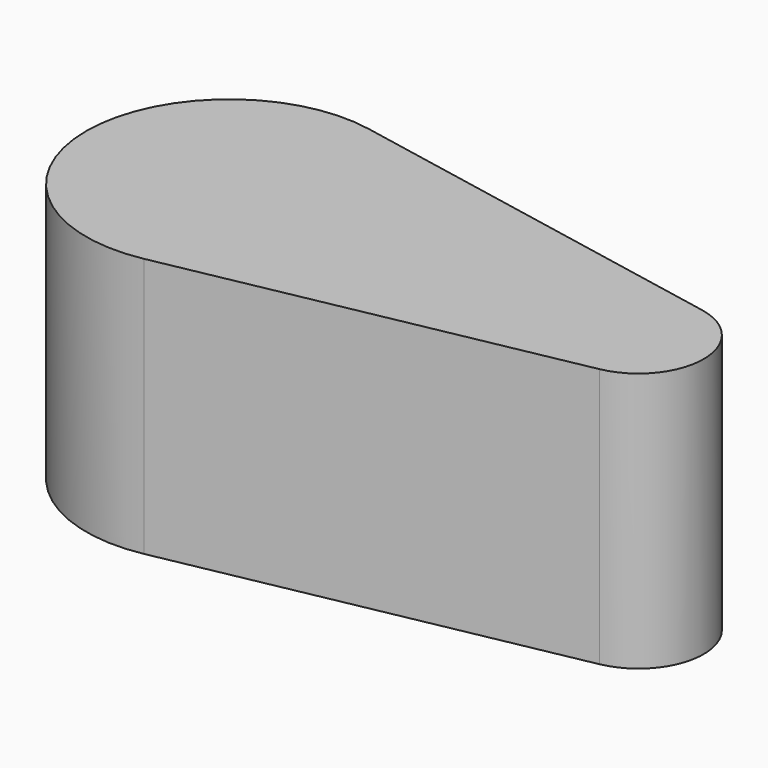
from build123d import *

# Parameters (mm, degrees)
F1_DEPTH = 25.4


with BuildPart() as f1:
    # F0 (on Top) → F1 (new body)
    with BuildSketch(Plane.XY):
        with BuildLine():
            Line((41.2148971477, 6.2581892729), (2.6675960663, 13.7413451978))
            ThreePointArc((2.6675960663, 13.7413451978), (-13.9978797186, 0), (2.6675960663, -13.7413451978))
            Line((2.6675960663, -13.7413451978), (41.2148971477, -6.2581892729))
            ThreePointArc((41.2148971477, -6.2581892729), (46.3750222003, 0), (41.2148971477, 6.2581892729))
        make_face()
    extrude(amount=F1_DEPTH)


solid = f1.part
